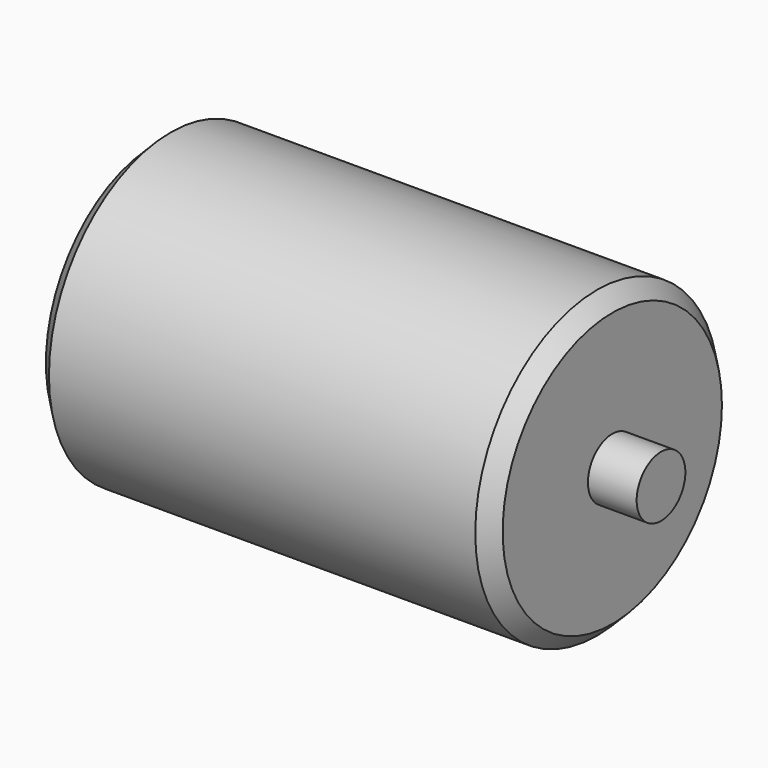
from build123d import *

# Parameters (mm, degrees)
F0_R     = 10
F1_DEPTH = 16
F0_R_2   = 50
F2_DEPTH = 150
F3_SIZE2 = 5
F3_SIZE  = 5
F4_SIZE2 = 5
F4_SIZE  = 5
F5_DEPTH = 166


with BuildPart() as f1:
    # F0 (on Right) → F1 (new body)
    with BuildSketch(Plane.YZ):
        Circle(F0_R)
    extrude(amount=F1_DEPTH)

    # F0 (on Right) → F5 (join)
    with BuildSketch(Plane.YZ):
        Circle(F0_R)
    extrude(amount=-F5_DEPTH)


with BuildPart() as f2:
    # F0 (on Right) → F2 (new body)
    with BuildSketch(Plane.YZ):
        Circle(F0_R_2)
        Circle(F0_R, mode=Mode.SUBTRACT)
    extrude(amount=-F2_DEPTH)

    # F3
    f3_edges = [f2.edges().sort_by_distance(p)[0] for p in [
        (0, -50, 0),
    ]]
    chamfer(f3_edges, length=F3_SIZE, length2=F3_SIZE2)

    # F4
    f4_edges = [f2.edges().sort_by_distance(p)[0] for p in [
        (-150, -50, 0),
    ]]
    chamfer(f4_edges, length=F4_SIZE, length2=F4_SIZE2)


solid = Compound([f1.part, f2.part])
